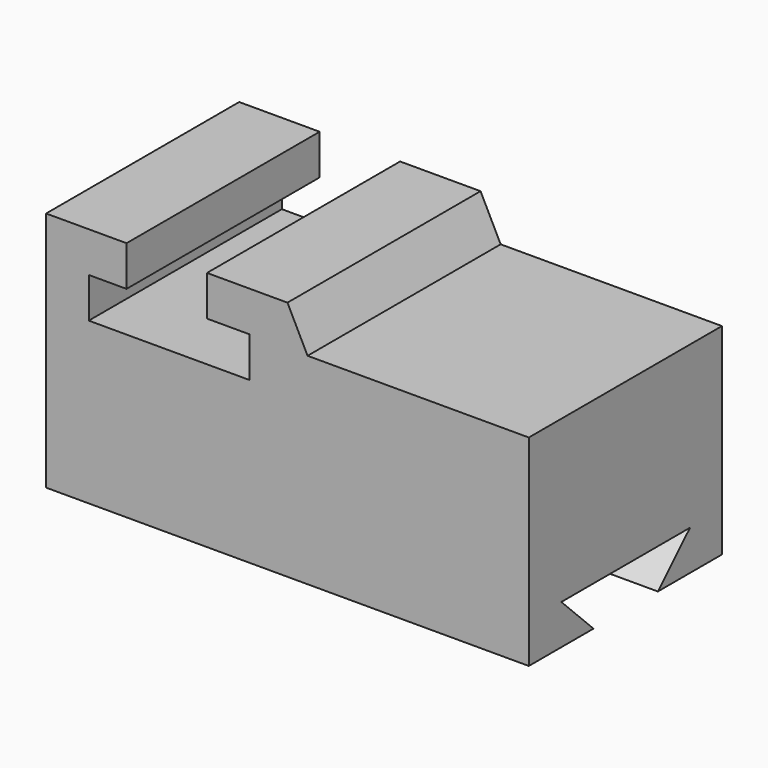
from build123d import *

# Parameters (mm, degrees)
F0_W      = 152.4
F0_H      = 76.2
F1_DEPTH  = 76.2
F3_DEPTH  = 152.4
F4_W      = 69.85
F4_H      = 12.7
F5_DEPTH  = 76.2
F7_DEPTH  = 76.2
F8_W      = 25.4
F8_H      = 12.7
F9_DEPTH  = 76.2
F11_DEPTH = 76.2


# Not quite as in the source:
# - a feature names something its author has since deleted; it is built from what else it names


with BuildPart() as f1:
    # F0 (on Front) → F1 (new body)
    with BuildSketch(Plane.XZ):
        with Locations((76.2, 38.1)):
            Rectangle(F0_W, F0_H)
    extrude(amount=-F1_DEPTH)

    # F2 (on face) → F3 (cut)
    with BuildSketch(Plane.YZ.offset(152.4)):
        Polygon((25.5270022899, 0), (38.1, 0), (50.9269982576, 0), (63.6270046234, 12.573000975), (12.8270015121, 12.573000975), align=None)
    extrude(amount=-F3_DEPTH, mode=Mode.SUBTRACT)

    # F4 (on face) → F5 (cut)
    with BuildSketch(Plane.XZ):
        with Locations((117.475, 69.85)):
            Rectangle(F4_W, F4_H)
    extrude(amount=-F5_DEPTH, mode=Mode.SUBTRACT)

    # F6 (on face) → F7 (cut)
    with BuildSketch(Plane.XZ):
        Polygon((76.2, 76.2), (82.55, 63.5), (82.55, 76.2), align=None)
    extrude(amount=-F7_DEPTH, mode=Mode.SUBTRACT)

    # F8 (on face) → F9 (cut)
    with BuildSketch(Plane.XZ):
        with Locations((38.1, 69.85)):
            Rectangle(F8_W, F8_H)
    extrude(amount=-F9_DEPTH, mode=Mode.SUBTRACT)

    # F10 (on face) → F11 (cut)
    with BuildSketch(Plane.XZ):
        Polygon((64.2725850075, 63.5), (38.1, 63.5), (13.4725850075, 63.5), (13.4725850075, 50.8), (64.2725850075, 50.8), align=None)
    extrude(amount=-F11_DEPTH, mode=Mode.SUBTRACT)


solid = f1.part
